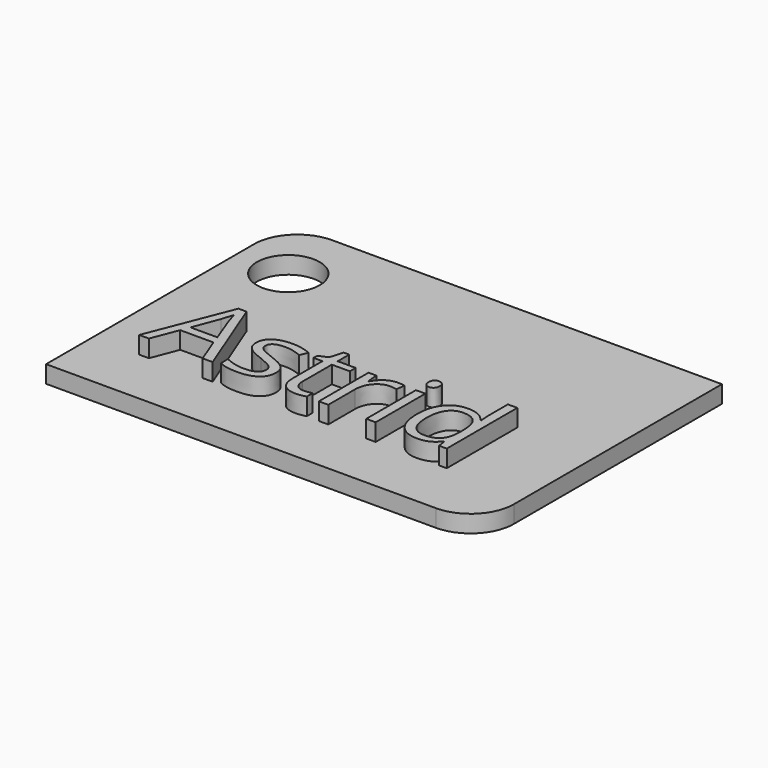
from build123d import *

# Parameters (mm, degrees)
F0_W         = 50
F0_H         = 35
F0_R         = 3.6268758291
F1_DEPTH     = 2
F2_R         = 5
F3_R         = 5
F4_TEXT_SIZE = 13.3910876078
F5_DEPTH     = 2


# Not quite as in the source:
# - Text() gives the source's letters only with a copy of the font that has no kerning and outlines rounded to 1/6400 em; it was checked with that copy


with BuildPart() as f1:
    # F0 (on Top) → F1 (new body)
    with BuildSketch(Plane.XY):
        Rectangle(F0_W, F0_H)
        with Locations((-18.9937204123, 9.9350996315)):
            Circle(F0_R, mode=Mode.SUBTRACT)
    extrude(amount=F1_DEPTH)

    # F2
    f2_edges = [f1.edges().sort_by_distance(p)[0] for p in [
        (-25, 17.5, 1),
    ]]
    fillet(f2_edges, radius=F2_R)

    # F3
    f3_edges = [f1.edges().sort_by_distance(p)[0] for p in [
        (25, -17.5, 1),
    ]]
    fillet(f3_edges, radius=F3_R)

    # F4 (on face) → F5 (join)
    with BuildSketch(Plane.XY.offset(2)):
        with Locations((-19.6112231351, -10.8062607469)):
            Text('Astrid', F4_TEXT_SIZE, font='Open Sans', text_align=(TextAlign.LEFT, TextAlign.BOTTOM))
    extrude(amount=F5_DEPTH)


solid = f1.part
